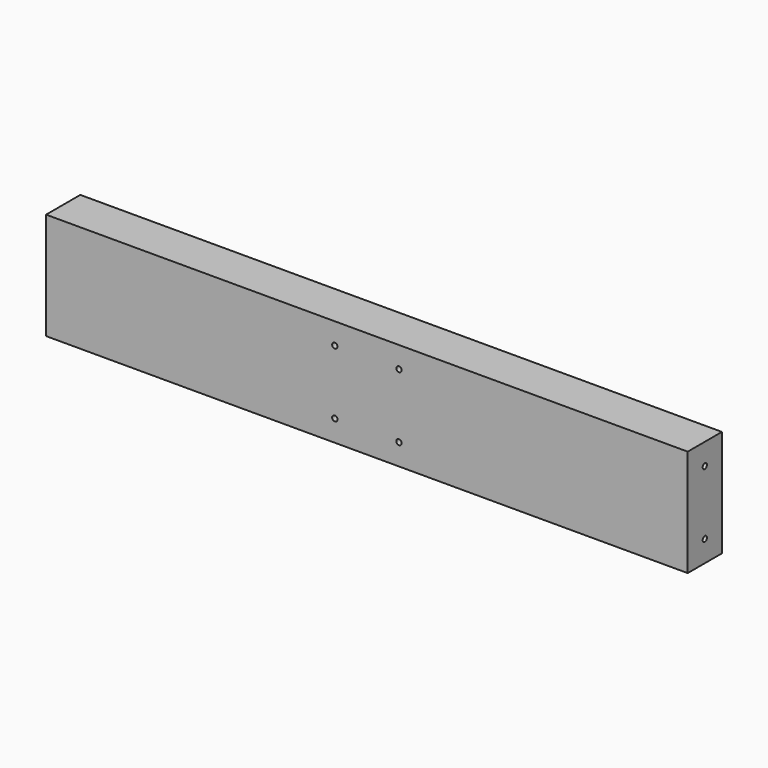
from build123d import *

# Parameters (mm, degrees)
F0_W     = 600
F0_H     = 100
F1_DEPTH = 20
F3_D     = 5
F5_D     = 5
F5_DEPTH = 50
F5_TIP   = 1.5021515476


# Not quite as in the source:
# - a feature names something its author has since deleted; it is built from what else it names


with BuildPart() as f1:
    # F0 (on Front) → F1 (new body, symmetric)
    with BuildSketch(Plane.XZ):
        Rectangle(F0_W, F0_H)
    extrude(amount=F1_DEPTH, both=True)

    # F3 (through all)
    with Locations(Plane.XZ.offset(20)):
        with Locations((-30, 30), (30, 30), (-30, -30), (30, -30)):
            Hole(F3_D / 2)

    # F5
    with Locations(Plane.YZ.offset(300)):
        with Locations((0, 30), (0, -30)):
            Hole(F5_D / 2, depth=F5_DEPTH)
            with Locations((0, 0, -(F5_DEPTH + F5_TIP / 2))):  # 118° drill point
                Cone(0, F5_D / 2, F5_TIP, mode=Mode.SUBTRACT)


solid = f1.part
